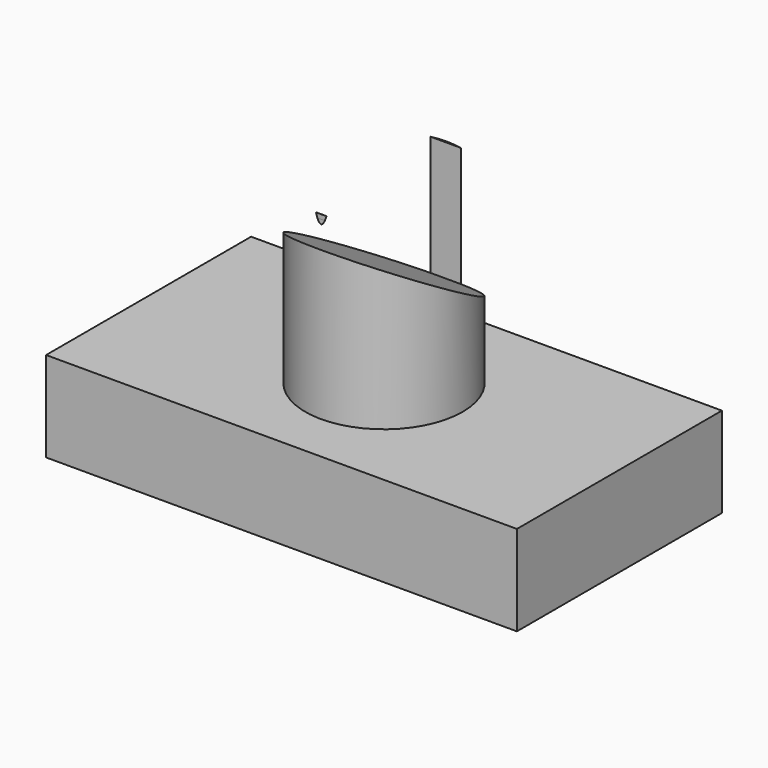
from build123d import *

# Parameters (mm, degrees)
F0_W          = 132.6039880514
F0_H          = 72.1768513322
F1_DEPTH      = 25.4
F2_R          = 22.1558784723
F3_DEPTH      = 50.8
F5_DEPTH      = 25.4
F5_DEPTH_BACK = 25.4


with BuildPart() as f1:
    # F0 (on Top) → F1 (new body)
    with BuildSketch(Plane.XY):
        Rectangle(F0_W, F0_H)
    extrude(amount=F1_DEPTH)

    # F2 (on face) → F3 (join)
    with BuildSketch(Plane.XY.offset(25.4)):
        Circle(F2_R)
    extrude(amount=F3_DEPTH)

    # F4 (on Right) → F5 (cut, two sides)
    with BuildSketch(Plane.YZ) as f5_sk:
        Polygon((-22.1006646752, 76.3731822371), (-22.2871676087, 67.4210116267), (21.7276569456, 42.4295440316), (21.7276569456, 76.3731822371), align=None)
    extrude(amount=-F5_DEPTH, mode=Mode.SUBTRACT)
    extrude(f5_sk.sketch, amount=F5_DEPTH_BACK, mode=Mode.SUBTRACT)


solid = f1.part
